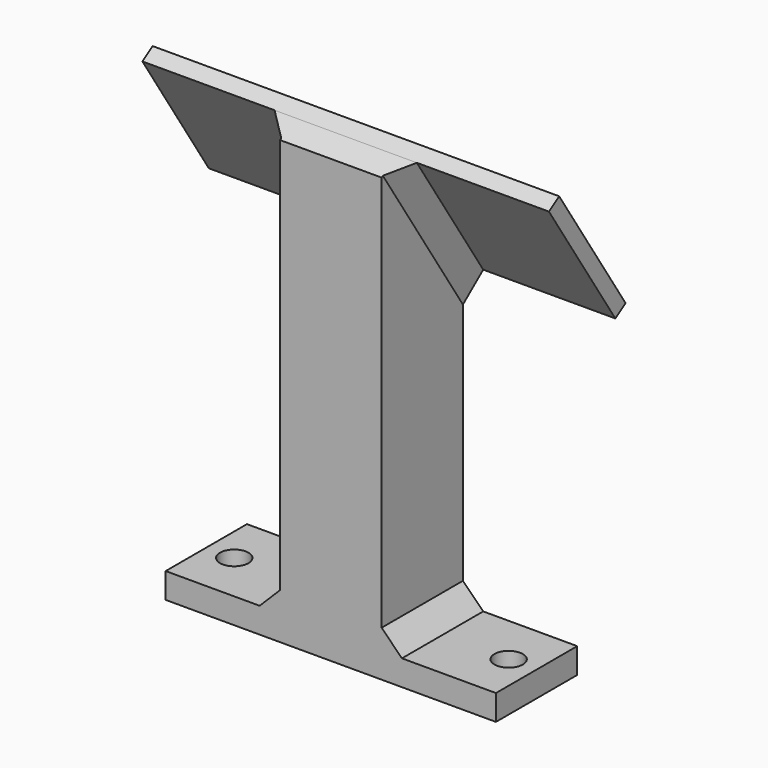
from build123d import *

# Parameters (mm, degrees)
F0_W     = 82.55
F0_H     = 25.4
F0_R     = 3.556
F1_DEPTH = 6.35
F2_W     = 25.4
F2_H     = 25.4
F3_DEPTH = 114.3
F5_DEPTH = 25.4
F6_W     = 38.1
F6_H     = 38.1
F6_W_2   = 25.4
F7_DEPTH = 3.81
F9_DEPTH = 25.4
F10_SIZE = 5.08


with BuildPart() as f1:
    # F0 (on Top) → F1 (new body)
    with BuildSketch(Plane.XY):
        Rectangle(F0_W, F0_H)
        with Locations((-34.29, 0)):
            Circle(F0_R, mode=Mode.SUBTRACT)
        with Locations((34.29, 0)):
            Circle(F0_R, mode=Mode.SUBTRACT)
    extrude(amount=F1_DEPTH)

    # F2 (on face) → F3 (join)
    with BuildSketch(Plane.XY.offset(6.35)):
        Rectangle(F2_W, F2_H)
    extrude(amount=F3_DEPTH)

    # F4 (on face) → F5 (cut)
    with BuildSketch(Plane.YZ.offset(12.7)):
        Polygon((12.7, 120.65), (-12.7, 120.65), (12.7, 81.5374299191), align=None)
    extrude(amount=-F5_DEPTH, mode=Mode.SUBTRACT)

    # F6 (on face) → F7 (join)
    with BuildSketch(Plane(origin=(0, 46.1768520488, 29.9875983504), x_dir=(-1, 0, 0), z_dir=(0, 0.8386705679, 0.544639035))):
        with Locations((-31.75, 80.5161269144)):
            Rectangle(F6_W, F6_H)
        with Locations((0, 80.5161269144)):
            Rectangle(F6_W_2, F6_H)
        with Locations((31.75, 80.5161269144)):
            Rectangle(F6_W, F6_H)
    extrude(amount=F7_DEPTH)

    # F8 (on face) → F9 (cut)
    with BuildSketch(Plane.YZ.offset(12.7)):
        Polygon((-12.7, 110.4715185089), (-8.0507472341, 113.4907785578), (-12.7, 120.65), align=None)
    extrude(amount=-F9_DEPTH, mode=Mode.SUBTRACT)

    # F10
    f10_edges = [f1.edges().sort_by_distance(p)[0] for p in [
        (12.7, 0, 6.35),
        (-12.7, 0, 6.35),
        (12.7, 2.324626, 97.514104),
        (-12.7, 2.324626, 97.514104),
    ]]
    chamfer(f10_edges, length=F10_SIZE)


solid = f1.part
